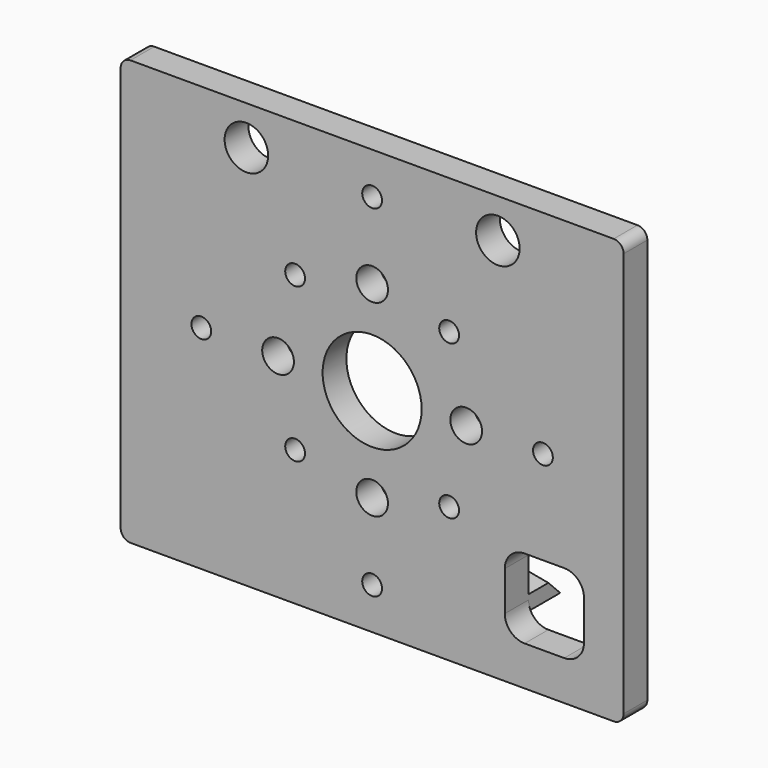
from build123d import *

# Parameters (mm, degrees)
F0_W     = 50.8
F0_H     = 42.9
F0_R     = 1
F0_R_2   = 1.6
F0_R_3   = 5
F0_R_4   = 2.2
F1_DEPTH = 3
F2_R     = 1
F3_W     = 3
F3_H     = 5
F3_H_2   = 4
F3_W_2   = 5
F3_H_3   = 3
F4_DEPTH = 4
F5_SIZE  = 1.5
F6_SIZE  = 2.99999
F7_SIZE  = 2.99999


# Not quite as in the source:
# - a fillet or chamfer is up to 0.001 mm smaller than in the source, because OpenCascade refuses the exact size


with BuildPart() as f1:
    # F0 (on Front) → F1 (new body)
    with BuildSketch(Plane.XZ):
        Rectangle(F0_W, F0_H)
        with Locations((0, -17.25)):
            Circle(F0_R, mode=Mode.SUBTRACT)
        with Locations((-7.7781745931, -7.7781745931)):
            Circle(F0_R, mode=Mode.SUBTRACT)
        with Locations((0, -9.5)):
            Circle(F0_R_2, mode=Mode.SUBTRACT)
        with BuildLine():
            ThreePointArc((21.4, -15.45), (20.8142135624, -16.8642135624), (19.4, -17.45))
            Line((19.4, -17.45), (15.4, -17.45))
            ThreePointArc((15.4, -17.45), (13.9857864376, -16.8642135624), (13.4, -15.45))
            Line((13.4, -15.45), (13.4, -11.45))
            ThreePointArc((13.4, -11.45), (13.9857864376, -10.0357864376), (15.4, -9.45))
            Line((15.4, -9.45), (19.4, -9.45))
            ThreePointArc((19.4, -9.45), (20.8142135624, -10.0357864376), (21.4, -11.45))
            Line((21.4, -11.45), (21.4, -15.45))
        make_face(mode=Mode.SUBTRACT)
        with Locations((7.7781745931, -7.7781745931)):
            Circle(F0_R, mode=Mode.SUBTRACT)
        with Locations((-17.25, 0)):
            Circle(F0_R, mode=Mode.SUBTRACT)
        with Locations((-9.5, 0)):
            Circle(F0_R_2, mode=Mode.SUBTRACT)
        Circle(F0_R_3, mode=Mode.SUBTRACT)
        with Locations((-7.7781745931, 7.7781745931)):
            Circle(F0_R, mode=Mode.SUBTRACT)
        with Locations((0, 9.5)):
            Circle(F0_R_2, mode=Mode.SUBTRACT)
        with Locations((-12.7, 17.5)):
            Circle(F0_R_4, mode=Mode.SUBTRACT)
        with Locations((0, 17.25)):
            Circle(F0_R, mode=Mode.SUBTRACT)
        with Locations((9.5, 0)):
            Circle(F0_R_2, mode=Mode.SUBTRACT)
        with Locations((7.7781745931, 7.7781745931)):
            Circle(F0_R, mode=Mode.SUBTRACT)
        with Locations((17.25, 0)):
            Circle(F0_R, mode=Mode.SUBTRACT)
        with Locations((12.7, 17.5)):
            Circle(F0_R_4, mode=Mode.SUBTRACT)
    extrude(amount=F1_DEPTH)

    # F2
    f2_edges = [f1.edges().sort_by_distance(p)[0] for p in [
        (25.4, -1.5, 21.45),
        (25.4, -1.5, -21.45),
        (-25.4, -1.5, -21.45),
        (-25.4, -1.5, 21.45),
    ]]
    fillet(f2_edges, radius=F2_R)

    # F3 (on face) → F4 (join)
    with BuildSketch(Plane(origin=(0, 0, 0), x_dir=(-1, 0, 0), z_dir=(0, 1, 0))):
        with Locations((-18.9, 13.95)):
            Rectangle(F3_W, F3_H)
        with Locations((-18.9, -7.45)):
            Rectangle(F3_W, F3_H_2)
        with Locations((18.9, 13.95)):
            Rectangle(F3_W, F3_H)
        Polygon((20.4, -16.45), (20.4, -5.45), (17.4, -5.45), (17.4, -13.45), (8.4, -13.45), (8.4, -16.45), align=None)
        with Locations((-10.9, -14.95)):
            Rectangle(F3_W_2, F3_H_3)
    extrude(amount=F4_DEPTH)

    # F5
    f5_edges = [f1.edges().sort_by_distance(p)[0] for p in [
        (13.4, 2, -13.45),
        (17.4, 2, -9.45),
    ]]
    chamfer(f5_edges, length=F5_SIZE)

    # F6 (size 3 in the source; OpenCascade refuses exactly that, so slightly less here)
    f6_edges = [f1.edges().sort_by_distance(p)[0] for p in [
        (17.4, 4, 13.95),
    ]]
    chamfer(f6_edges, length=F6_SIZE)

    # F7 (size 3 in the source; OpenCascade refuses exactly that, so slightly less here)
    f7_edges = [f1.edges().sort_by_distance(p)[0] for p in [
        (-17.4, 4, 13.95),
        (-17.4, 4, -9.45),
        (-12.9, 4, -13.45),
        (10.15, 4, -13.45),
        (17.4, 4, -6.7),
    ]]
    chamfer(f7_edges, length=F7_SIZE)


solid = f1.part
